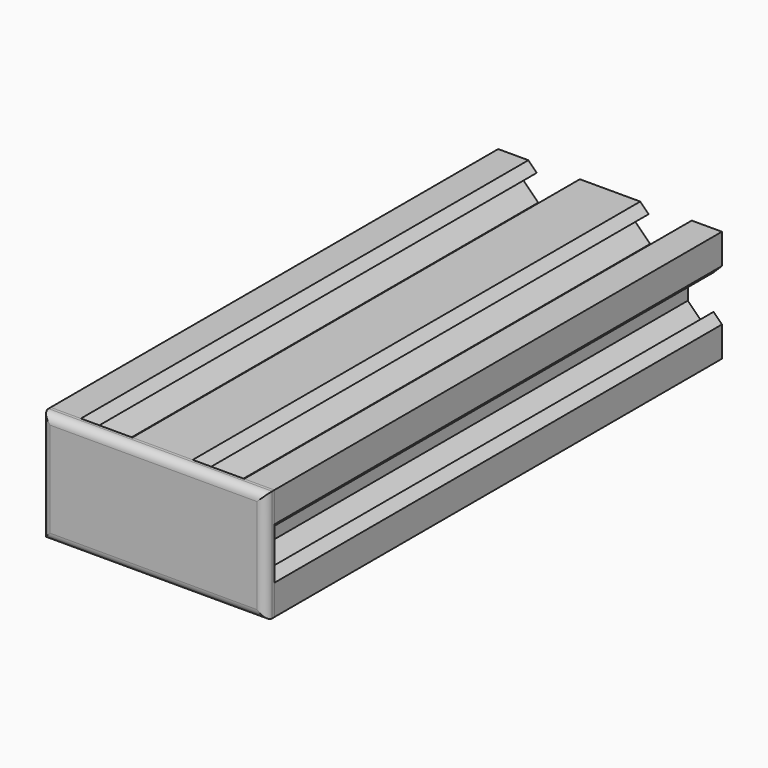
from build123d import *

# Parameters (mm, degrees)
F1_DEPTH      = 50
F3_DEPTH      = 2
F4_W          = 38.4
F4_H          = 18.3999997326
F5_DEPTH      = 0.6
F6_DEPTH      = 4
F6_DEPTH_BACK = 1
F7_R          = 1.5


with BuildPart() as f1:
    # F0 (on Front) → F1 (new body, symmetric)
    with BuildSketch(Plane.XZ):
        Polygon((-15.5, 6.5606601718), (-15.5, 8.4999998663), (-13.1, 8.4999998663), (-14.6, 9.9999998663), (-20, 9.9999998663), (-20, 4.5999998663), (-18.4999998663, 3.1), (-18.4999998663, 5.5), (-16.5606601718, 5.5), (-13.9, 2.8393398282), (-13.9, 0.1), (-13.7, 0.1), (-13.7, 0), (-13.7, -0.1), (-13.9, -0.1), (-13.9, -2.8393398282), (-16.5606601718, -5.5), (-18.4999998663, -5.5), (-18.4999998663, -3.1), (-20, -4.5999998663), (-20, -9.9999998663), (-14.6, -9.9999998663), (-13.1, -8.4999998663), (-15.5, -8.4999998663), (-15.5, -6.5606601718), (-12.8393398282, -3.9), (-10.1, -3.9), (-10.1, -3.7), (-9.9, -3.7), (-9.9, -3.9), (-7.1606601718, -3.9), (-4.5, -6.5606601718), (-4.5, -8.4999998663), (-6.9, -8.4999998663), (-5.4, -9.9999998663), (0, -9.9999998663), (5.4, -9.9999998663), (6.9, -8.4999998663), (4.5, -8.4999998663), (4.5, -6.5606601718), (7.1606601718, -3.9), (9.9, -3.9), (9.9, -3.7), (10.1, -3.7), (10.1, -3.9), (12.8393398282, -3.9), (15.5, -6.5606601718), (15.5, -8.4999998663), (13.1, -8.4999998663), (14.6, -9.9999998663), (20, -9.9999998663), (20, -4.5999998663), (18.4999998663, -3.1), (18.4999998663, -5.5), (16.5606601718, -5.5), (13.9, -2.8393398282), (13.9, -0.1), (13.7, -0.1), (13.7, 0), (13.7, 0.1), (13.9, 0.1), (13.9, 2.8393398282), (16.5606601718, 5.5), (18.4999998663, 5.5), (18.4999998663, 3.1), (20, 4.5999998663), (20, 9.9999998663), (14.6, 9.9999998663), (13.1, 8.4999998663), (15.5, 8.4999998663), (15.5, 6.5606601718), (12.8393398282, 3.9), (10.1, 3.9), (10.1, 3.7), (9.9, 3.7), (9.9, 3.9), (7.1606601718, 3.9), (4.5, 6.5606601718), (4.5, 8.4999998663), (6.9, 8.4999998663), (5.4, 9.9999998663), (0, 9.9999998663), (-5.4, 9.9999998663), (-6.9, 8.4999998663), (-4.5, 8.4999998663), (-4.5, 6.5606601718), (-7.1606601718, 3.9), (-9.9, 3.9), (-9.9, 3.7), (-10.1, 3.7), (-10.1, 3.9), (-12.8393398282, 3.9), align=None)
        with BuildLine():
            ThreePointArc((-12.1, 0), (-10, 2.1), (-7.9, 0))
            ThreePointArc((-7.9, 0), (-10, -2.1), (-12.1, 0))
        make_face(mode=Mode.SUBTRACT)
        Polygon((-6.1, 2.8393398282), (-2.8, 6.1393398282), (-2.8, 8.4999998663), (0, 8.4999998663), (2.8, 8.4999998663), (2.8, 6.1393398282), (6.1, 2.8393398282), (6.1, 0), (6.1, -2.8393398282), (2.8, -6.1393398282), (2.8, -8.4999998663), (0, -8.4999998663), (-2.8, -8.4999998663), (-2.8, -6.1393398282), (-6.1, -2.8393398282), (-6.1, 0), align=None, mode=Mode.SUBTRACT)
        with BuildLine():
            ThreePointArc((12.1, 0), (10, -2.1), (7.9, 0))
            ThreePointArc((7.9, 0), (10, 2.1), (12.1, 0))
        make_face(mode=Mode.SUBTRACT)
    extrude(amount=F1_DEPTH, both=True)


with BuildPart() as f3:
    # F2 (on face) → F3 (new body)
    with BuildSketch(Plane.XZ.offset(50)):
        Polygon((-14.6, 9.9999998663), (-20, 9.9999998663), (-20, 4.5999998663), (-18.4999998663, 3.1), (-18.4999998663, 5.5), (-16.5606601718, 5.5), (-13.9, 2.8393398282), (-13.9, 0.1), (-13.7, 0.1), (-13.7, -0.1), (-13.9, -0.1), (-13.9, -2.8393398282), (-16.5606601718, -5.5), (-18.4999998663, -5.5), (-18.4999998663, -3.1), (-20, -4.5999998663), (-20, -9.9999998663), (-14.6, -9.9999998663), (-13.1, -8.4999998663), (-15.5, -8.4999998663), (-15.5, -6.5606601718), (-12.8393398282, -3.9), (-10.1, -3.9), (-10.1, -3.7), (-9.9, -3.7), (-9.9, -3.9), (-7.1606601718, -3.9), (-4.5, -6.5606601718), (-4.5, -8.4999998663), (-6.9, -8.4999998663), (-5.4, -9.9999998663), (5.4, -9.9999998663), (6.9, -8.4999998663), (4.5, -8.4999998663), (4.5, -6.5606601718), (7.1606601718, -3.9), (9.9, -3.9), (9.9, -3.7), (10.1, -3.7), (10.1, -3.9), (12.8393398282, -3.9), (15.5, -6.5606601718), (15.5, -8.4999998663), (13.1, -8.4999998663), (14.6, -9.9999998663), (20, -9.9999998663), (20, -4.5999998663), (18.4999998663, -3.1), (18.4999998663, -5.5), (16.5606601718, -5.5), (13.9, -2.8393398282), (13.9, -0.1), (13.7, -0.1), (13.7, 0.1), (13.9, 0.1), (13.9, 2.8393398282), (16.5606601718, 5.5), (18.4999998663, 5.5), (18.4999998663, 3.1), (20, 4.5999998663), (20, 9.9999998663), (14.6, 9.9999998663), (13.1, 8.4999998663), (15.5, 8.4999998663), (15.5, 6.5606601718), (12.8393398282, 3.9), (10.1, 3.9), (10.1, 3.7), (9.9, 3.7), (9.9, 3.9), (7.1606601718, 3.9), (4.5, 6.5606601718), (4.5, 8.4999998663), (6.9, 8.4999998663), (5.4, 9.9999998663), (-5.4, 9.9999998663), (-6.9, 8.4999998663), (-4.5, 8.4999998663), (-4.5, 6.5606601718), (-7.1606601718, 3.9), (-9.9, 3.9), (-9.9, 3.7), (-10.1, 3.7), (-10.1, 3.9), (-12.8393398282, 3.9), (-15.5, 6.5606601718), (-15.5, 8.4999998663), (-13.1, 8.4999998663), align=None)
        with BuildLine():
            ThreePointArc((-9.8, 2.090454496), (-8.4459729732, 1.4124446892), (-7.9, 0))
            ThreePointArc((-7.9, 0), (-8.4459729732, -1.4124446892), (-9.8, -2.090454496))
            ThreePointArc((-9.8, -2.090454496), (-10, -2.1), (-10.2, -2.090454496))
            ThreePointArc((-10.2, -2.090454496), (-11.5540270268, -1.4124446892), (-12.1, 0))
            ThreePointArc((-12.1, 0), (-11.5540270268, 1.4124446892), (-10.2, 2.090454496))
            ThreePointArc((-10.2, 2.090454496), (-10, 2.1), (-9.8, 2.090454496))
        make_face(mode=Mode.SUBTRACT)
        Polygon((6.1, -2.8393398282), (2.8, -6.1393398282), (2.8, -8.4999998663), (0, -8.4999998663), (-2.8, -8.4999998663), (-2.8, -6.1393398282), (-6.1, -2.8393398282), (-6.1, 0), (-6.1, 2.8393398282), (-2.8, 6.1393398282), (-2.8, 8.4999998663), (0, 8.4999998663), (2.8, 8.4999998663), (2.8, 6.1393398282), (6.1, 2.8393398282), (6.1, 0), align=None, mode=Mode.SUBTRACT)
        with BuildLine():
            ThreePointArc((10.2, 2.090454496), (11.5540270268, 1.4124446892), (12.1, 0))
            ThreePointArc((12.1, 0), (11.5540270268, -1.4124446892), (10.2, -2.090454496))
            ThreePointArc((10.2, -2.090454496), (10, -2.1), (9.8, -2.090454496))
            ThreePointArc((9.8, -2.090454496), (8.4459729732, -1.4124446892), (7.9, 0))
            ThreePointArc((7.9, 0), (8.4459729732, 1.4124446892), (9.8, 2.090454496))
            ThreePointArc((9.8, 2.090454496), (10, 2.1), (10.2, 2.090454496))
        make_face(mode=Mode.SUBTRACT)
        Polygon((2.8, -8.4999998663), (2.8, -6.1393398282), (6.1, -2.8393398282), (6.1, 0), (6.1, 2.8393398282), (2.8, 6.1393398282), (2.8, 8.4999998663), (0, 8.4999998663), (-2.8, 8.4999998663), (-2.8, 6.1393398282), (-6.1, 2.8393398282), (-6.1, 0), (-6.1, -2.8393398282), (-2.8, -6.1393398282), (-2.8, -8.4999998663), (0, -8.4999998663), align=None)
        Polygon((20, -4.5999998663), (20, 4.5999998663), (18.4999998663, 3.1), (18.4999998663, 5.5), (16.5606601718, 5.5), (13.9, 2.8393398282), (13.9, 0.1), (13.7, 0.1), (13.7, -0.1), (13.9, -0.1), (13.9, -2.8393398282), (16.5606601718, -5.5), (18.4999998663, -5.5), (18.4999998663, -3.1), align=None)
        Polygon((-18.4999998663, 3.1), (-20, 4.5999998663), (-20, -4.5999998663), (-18.4999998663, -3.1), (-18.4999998663, -5.5), (-16.5606601718, -5.5), (-13.9, -2.8393398282), (-13.9, -0.1), (-13.7, -0.1), (-13.7, 0.1), (-13.9, 0.1), (-13.9, 2.8393398282), (-16.5606601718, 5.5), (-18.4999998663, 5.5), align=None)
        Polygon((-5.4, 9.9999998663), (-14.6, 9.9999998663), (-13.1, 8.4999998663), (-15.5, 8.4999998663), (-15.5, 6.5606601718), (-12.8393398282, 3.9), (-10.1, 3.9), (-10.1, 3.7), (-9.9, 3.7), (-9.9, 3.9), (-7.1606601718, 3.9), (-4.5, 6.5606601718), (-4.5, 8.4999998663), (-6.9, 8.4999998663), align=None)
        Polygon((14.6, 9.9999998663), (5.4, 9.9999998663), (6.9, 8.4999998663), (4.5, 8.4999998663), (4.5, 6.5606601718), (7.1606601718, 3.9), (9.9, 3.9), (9.9, 3.7), (10.1, 3.7), (10.1, 3.9), (12.8393398282, 3.9), (15.5, 6.5606601718), (15.5, 8.4999998663), (13.1, 8.4999998663), align=None)
        Polygon((6.9, -8.4999998663), (5.4, -9.9999998663), (14.6, -9.9999998663), (13.1, -8.4999998663), (15.5, -8.4999998663), (15.5, -6.5606601718), (12.8393398282, -3.9), (10.1, -3.9), (10.1, -3.7), (9.9, -3.7), (9.9, -3.9), (7.1606601718, -3.9), (4.5, -6.5606601718), (4.5, -8.4999998663), align=None)
        Polygon((-13.1, -8.4999998663), (-14.6, -9.9999998663), (-5.4, -9.9999998663), (-6.9, -8.4999998663), (-4.5, -8.4999998663), (-4.5, -6.5606601718), (-7.1606601718, -3.9), (-9.9, -3.9), (-9.9, -3.7), (-10.1, -3.7), (-10.1, -3.9), (-12.8393398282, -3.9), (-15.5, -6.5606601718), (-15.5, -8.4999998663), align=None)
        with BuildLine():
            ThreePointArc((-8.3, 0), (-8.7291734973, 1.1291589791), (-9.8, 1.6881943016))
            ThreePointArc((-9.8, 1.6881943016), (-10, 1.7), (-10.2, 1.6881943016))
            ThreePointArc((-10.2, 1.6881943016), (-11.7, 0), (-10.2, -1.6881943016))
            ThreePointArc((-10.2, -1.6881943016), (-10, -1.7), (-9.8, -1.6881943016))
            ThreePointArc((-9.8, -1.6881943016), (-8.7291734973, -1.1291589791), (-8.3, 0))
        make_face()
        with BuildLine():
            ThreePointArc((11.7, 0), (11.2708265027, 1.1291589791), (10.2, 1.6881943016))
            ThreePointArc((10.2, 1.6881943016), (10, 1.7), (9.8, 1.6881943016))
            ThreePointArc((9.8, 1.6881943016), (8.3, 0), (9.8, -1.6881943016))
            ThreePointArc((9.8, -1.6881943016), (10, -1.7), (10.2, -1.6881943016))
            ThreePointArc((10.2, -1.6881943016), (11.2708265027, -1.1291589791), (11.7, 0))
        make_face()
        with BuildLine():
            Line((9.8, 1.6881943016), (9.8, 2.090454496))
            ThreePointArc((9.8, 2.090454496), (8.4459729732, 1.4124446892), (7.9, 0))
            ThreePointArc((7.9, 0), (8.4459729732, -1.4124446892), (9.8, -2.090454496))
            Line((9.8, -2.090454496), (9.8, -1.6881943016))
            ThreePointArc((9.8, -1.6881943016), (8.3, 0), (9.8, 1.6881943016))
        make_face()
        with BuildLine():
            ThreePointArc((10.2, -2.090454496), (11.5540270268, -1.4124446892), (12.1, 0))
            ThreePointArc((12.1, 0), (11.5540270268, 1.4124446892), (10.2, 2.090454496))
            Line((10.2, 2.090454496), (10.2, 1.6881943016))
            ThreePointArc((10.2, 1.6881943016), (11.2708265027, 1.1291589791), (11.7, 0))
            ThreePointArc((11.7, 0), (11.2708265027, -1.1291589791), (10.2, -1.6881943016))
            Line((10.2, -1.6881943016), (10.2, -2.090454496))
        make_face()
        with BuildLine():
            Line((-10.2, 1.6881943016), (-10.2, 2.090454496))
            ThreePointArc((-10.2, 2.090454496), (-11.5540270268, 1.4124446892), (-12.1, 0))
            ThreePointArc((-12.1, 0), (-11.5540270268, -1.4124446892), (-10.2, -2.090454496))
            Line((-10.2, -2.090454496), (-10.2, -1.6881943016))
            ThreePointArc((-10.2, -1.6881943016), (-11.7, 0), (-10.2, 1.6881943016))
        make_face()
        with BuildLine():
            ThreePointArc((-9.8, -2.090454496), (-8.4459729732, -1.4124446892), (-7.9, 0))
            ThreePointArc((-7.9, 0), (-8.4459729732, 1.4124446892), (-9.8, 2.090454496))
            Line((-9.8, 2.090454496), (-9.8, 1.6881943016))
            ThreePointArc((-9.8, 1.6881943016), (-8.7291734973, 1.1291589791), (-8.3, 0))
            ThreePointArc((-8.3, 0), (-8.7291734973, -1.1291589791), (-9.8, -1.6881943016))
            Line((-9.8, -1.6881943016), (-9.8, -2.090454496))
        make_face()
        with BuildLine():
            Line((10.2, 1.6881943016), (10.2, 2.090454496))
            ThreePointArc((10.2, 2.090454496), (10, 2.1), (9.8, 2.090454496))
            Line((9.8, 2.090454496), (9.8, 1.6881943016))
            ThreePointArc((9.8, 1.6881943016), (10, 1.7), (10.2, 1.6881943016))
        make_face()
        with BuildLine():
            ThreePointArc((9.8, -2.090454496), (10, -2.1), (10.2, -2.090454496))
            Line((10.2, -2.090454496), (10.2, -1.6881943016))
            ThreePointArc((10.2, -1.6881943016), (10, -1.7), (9.8, -1.6881943016))
            Line((9.8, -1.6881943016), (9.8, -2.090454496))
        make_face()
        with BuildLine():
            Line((-9.8, 1.6881943016), (-9.8, 2.090454496))
            ThreePointArc((-9.8, 2.090454496), (-10, 2.1), (-10.2, 2.090454496))
            Line((-10.2, 2.090454496), (-10.2, 1.6881943016))
            ThreePointArc((-10.2, 1.6881943016), (-10, 1.7), (-9.8, 1.6881943016))
        make_face()
        with BuildLine():
            ThreePointArc((-10.2, -2.090454496), (-10, -2.1), (-9.8, -2.090454496))
            Line((-9.8, -2.090454496), (-9.8, -1.6881943016))
            ThreePointArc((-9.8, -1.6881943016), (-10, -1.7), (-10.2, -1.6881943016))
            Line((-10.2, -1.6881943016), (-10.2, -2.090454496))
        make_face()
    extrude(amount=F3_DEPTH)

    # F4 (on face) → F5 (cut)
    with BuildSketch(Plane(origin=(0, -50, 0), x_dir=(-1, 0, 0), z_dir=(0, 1, 0))):
        Rectangle(F4_W, F4_H)
    extrude(amount=-F5_DEPTH, mode=Mode.SUBTRACT)

    # F2 (on face) → F6 (join, two sides)
    with BuildSketch(Plane.XZ.offset(50)) as f6_sk:
        with BuildLine():
            ThreePointArc((10.2, -2.090454496), (11.5540270268, -1.4124446892), (12.1, 0))
            ThreePointArc((12.1, 0), (11.5540270268, 1.4124446892), (10.2, 2.090454496))
            Line((10.2, 2.090454496), (10.2, 1.6881943016))
            ThreePointArc((10.2, 1.6881943016), (11.2708265027, 1.1291589791), (11.7, 0))
            ThreePointArc((11.7, 0), (11.2708265027, -1.1291589791), (10.2, -1.6881943016))
            Line((10.2, -1.6881943016), (10.2, -2.090454496))
        make_face()
        with BuildLine():
            Line((9.8, 1.6881943016), (9.8, 2.090454496))
            ThreePointArc((9.8, 2.090454496), (8.4459729732, 1.4124446892), (7.9, 0))
            ThreePointArc((7.9, 0), (8.4459729732, -1.4124446892), (9.8, -2.090454496))
            Line((9.8, -2.090454496), (9.8, -1.6881943016))
            ThreePointArc((9.8, -1.6881943016), (8.3, 0), (9.8, 1.6881943016))
        make_face()
        with BuildLine():
            ThreePointArc((-9.8, -2.090454496), (-8.4459729732, -1.4124446892), (-7.9, 0))
            ThreePointArc((-7.9, 0), (-8.4459729732, 1.4124446892), (-9.8, 2.090454496))
            Line((-9.8, 2.090454496), (-9.8, 1.6881943016))
            ThreePointArc((-9.8, 1.6881943016), (-8.7291734973, 1.1291589791), (-8.3, 0))
            ThreePointArc((-8.3, 0), (-8.7291734973, -1.1291589791), (-9.8, -1.6881943016))
            Line((-9.8, -1.6881943016), (-9.8, -2.090454496))
        make_face()
        with BuildLine():
            Line((-10.2, 1.6881943016), (-10.2, 2.090454496))
            ThreePointArc((-10.2, 2.090454496), (-11.5540270268, 1.4124446892), (-12.1, 0))
            ThreePointArc((-12.1, 0), (-11.5540270268, -1.4124446892), (-10.2, -2.090454496))
            Line((-10.2, -2.090454496), (-10.2, -1.6881943016))
            ThreePointArc((-10.2, -1.6881943016), (-11.7, 0), (-10.2, 1.6881943016))
        make_face()
    extrude(amount=-F6_DEPTH)
    extrude(f6_sk.sketch, amount=F6_DEPTH_BACK)

    # F7
    f7_edges = [f3.edges().sort_by_distance(p)[0] for p in [
        (0, -52, 10),
        (-20, -52, 0),
        (0, -52, -10),
        (20, -52, 0),
    ]]
    fillet(f7_edges, radius=F7_R)


solid = Compound([f1.part, f3.part])
